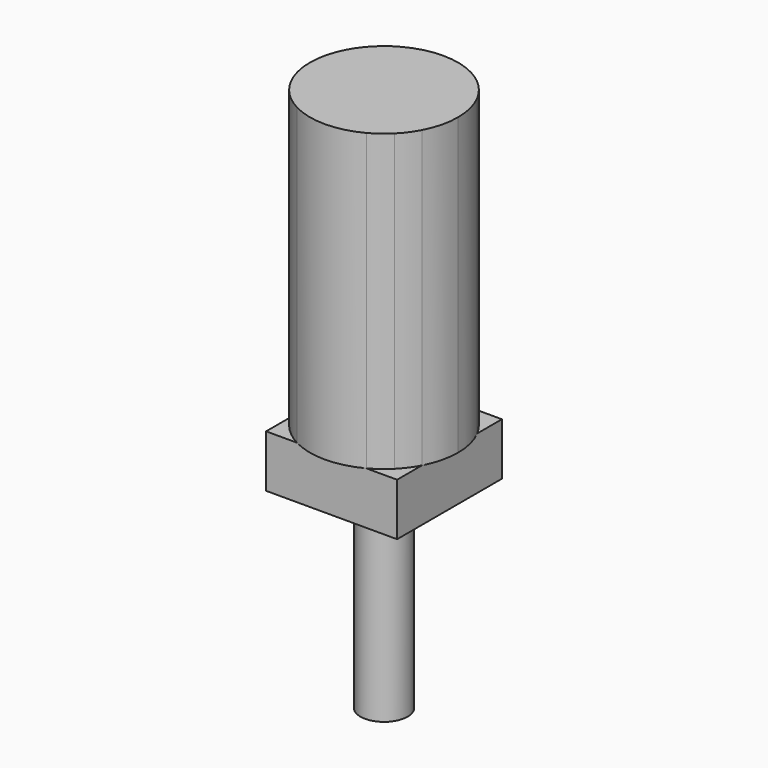
from build123d import *

# Parameters (mm, degrees)
F0_R     = 19.2528959131
F0_R_2   = 10
F1_DEPTH = 25
F0_W     = 50
F0_H     = 50
F0_W_2   = 40
F0_H_2   = 40
F2_DEPTH = 20
F3_R     = 9
F4_DEPTH = 100
F5_W     = 40
F5_H     = 40
F6_DEPTH = 112.7


with BuildPart() as f1:
    # F0 (on Top) → F1 (new body)
    with BuildSketch(Plane.XY):
        Circle(F0_R)
        Circle(F0_R_2, mode=Mode.SUBTRACT)
    extrude(amount=F1_DEPTH)


with BuildPart() as f2:
    # F0 (on Top) → F2 (new body)
    with BuildSketch(Plane.XY):
        Rectangle(F0_W, F0_H)
        Rectangle(F0_W_2, F0_H_2, mode=Mode.SUBTRACT)
    extrude(amount=F2_DEPTH)


with BuildPart() as f4:
    # F3 (on face) → F4 (new body)
    with BuildSketch(Plane.XY.offset(25)):
        Circle(F3_R)
    extrude(amount=-F4_DEPTH)


with BuildPart() as f6:
    # F5 (on face) → F6 (new body)
    with BuildSketch(Plane.XY.offset(20)):
        with BuildLine():
            ThreePointArc((25, -13.2287565553), (27.4509269533, -6.8151749359), (28.2842712475, 0))
            ThreePointArc((28.2842712475, 0), (27.4509269533, 6.8151749359), (25, 13.2287565553))
            Line((25, 13.2287565553), (25, -13.2287565553))
        make_face()
        with BuildLine():
            Line((25, -13.2287565553), (25, 13.2287565553))
            ThreePointArc((25, 13.2287565553), (22.7532950239, 16.8014155818), (20, 20))
            Line((20, 20), (20, -20))
            ThreePointArc((20, -20), (22.7532950239, -16.8014155818), (25, -13.2287565553))
        make_face()
        with BuildLine():
            Line((-20, 20), (20, 20))
            ThreePointArc((20, 20), (16.8014155818, 22.7532950239), (13.2287565553, 25))
            Line((13.2287565553, 25), (-13.2287565553, 25))
            ThreePointArc((-13.2287565553, 25), (-16.8014155818, 22.7532950239), (-20, 20))
        make_face()
        Rectangle(F5_W, F5_H)
        with BuildLine():
            ThreePointArc((13.2287565553, -25), (16.8014155818, -22.7532950239), (20, -20))
            Line((20, -20), (-20, -20))
            ThreePointArc((-20, -20), (-16.8014155818, -22.7532950239), (-13.2287565553, -25))
            Line((-13.2287565553, -25), (13.2287565553, -25))
        make_face()
        with BuildLine():
            Line((-13.2287565553, 25), (13.2287565553, 25))
            ThreePointArc((13.2287565553, 25), (0, 28.2842712475), (-13.2287565553, 25))
        make_face()
        with BuildLine():
            Line((-20, -20), (-20, 20))
            ThreePointArc((-20, 20), (-22.7532950239, 16.8014155818), (-25, 13.2287565553))
            Line((-25, 13.2287565553), (-25, -13.2287565553))
            ThreePointArc((-25, -13.2287565553), (-22.7532950239, -16.8014155818), (-20, -20))
        make_face()
        with BuildLine():
            ThreePointArc((-13.2287565553, -25), (0, -28.2842712475), (13.2287565553, -25))
            Line((13.2287565553, -25), (-13.2287565553, -25))
        make_face()
        with BuildLine():
            Line((-25, -13.2287565553), (-25, 13.2287565553))
            ThreePointArc((-25, 13.2287565553), (-28.2842712475, 0), (-25, -13.2287565553))
        make_face()
    extrude(amount=F6_DEPTH)


solid = Compound([f1.part, f2.part, f4.part, f6.part])
